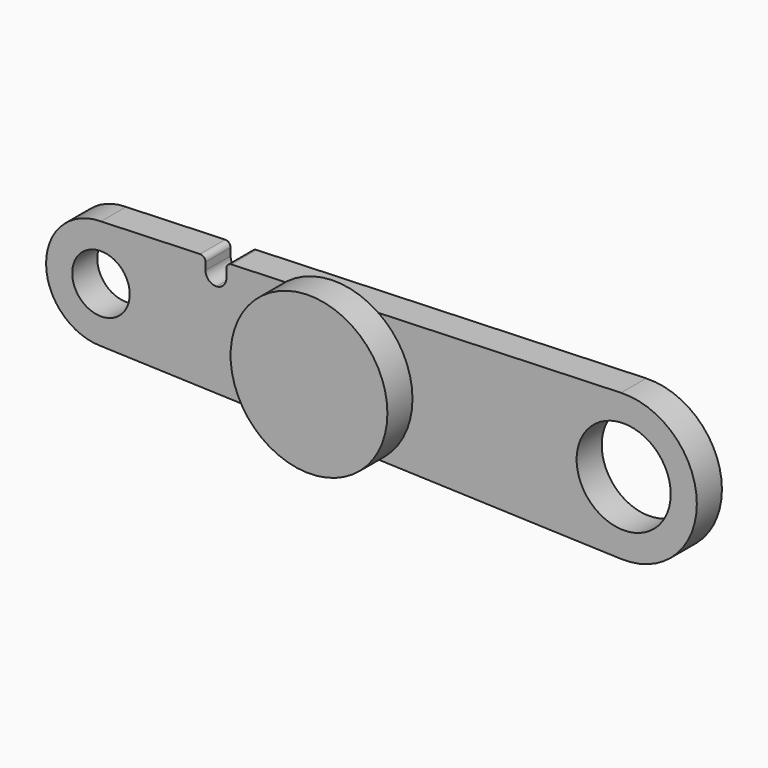
from build123d import *

# Parameters (mm, degrees)
F0_R     = 2.75
F0_R_2   = 4.5
F1_DEPTH = 3
F2_R     = 7.5
F3_DEPTH = 3


# Not quite as in the source:
# - a feature names something its author has since deleted; it is built from what else it names


with BuildPart() as f1:
    # F0 (on Front) → F1 (new body)
    with BuildSketch(Plane.XZ):
        with BuildLine():
            Line((-50, -5.25), (-0.2454519891, -6.9956953422))
            ThreePointArc((-0.2454519891, -6.9956953422), (7, 0), (-0.2454519891, 6.9956953422))
            Line((-0.2454519891, 6.9956953422), (-37.5175322849, 5.6879616863))
            ThreePointArc((-37.5175322849, 5.6879616863), (-37.8596985839, 5.5355686418), (-38, 5.1882691619))
            Line((-38, 5.1882691619), (-38, 4.3684233323))
            ThreePointArc((-38, 4.3684233323), (-38.2717414077, 3.6831209007), (-38.9392788456, 3.370268564))
            ThreePointArc((-38.9392788456, 3.370268564), (-39.6853024316, 3.6401647401), (-40, 4.3684233323))
            Line((-40, 4.3684233323), (-40, 5.0830107235))
            ThreePointArc((-40, 5.0830107235), (-40.1527005201, 5.4427093074), (-40.5175322849, 5.5827032479))
            Line((-40.5175322849, 5.5827032479), (-50, 5.25))
            ThreePointArc((-50, 5.25), (-55.25, 0), (-50, -5.25))
        make_face()
        with Locations((-50, 0)):
            Circle(F0_R, mode=Mode.SUBTRACT)
        Circle(F0_R_2, mode=Mode.SUBTRACT)
    extrude(amount=F1_DEPTH)


with BuildPart() as f3:
    # F2 (on Front) → F3 (new body)
    with BuildSketch(Plane.XZ):
        with Locations((-27.7, 0)):
            Circle(F2_R)
    extrude(amount=F3_DEPTH)


with BuildPart() as f3_1:
    # F4: moved
    add(f3.part.moved(Location((0, -3, 0))))


solid = Compound([f1.part, f3_1.part])
